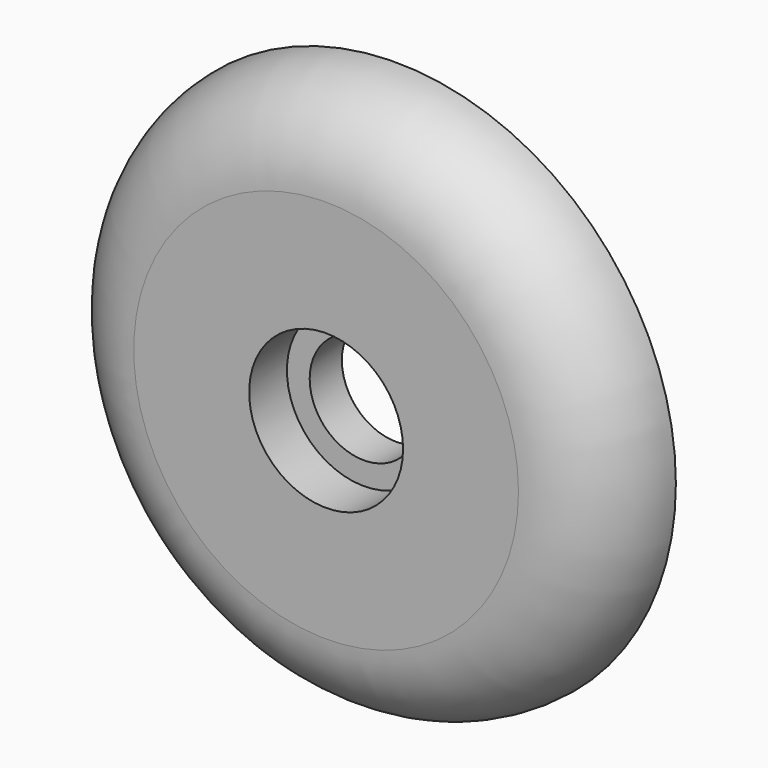
from build123d import *

# Parameters (mm, degrees)
F0_R     = 8
F1_DEPTH = 2.5
F2_R     = 2.49999
F3_R     = 1.55
F4_DEPTH = 25
F5_R     = 2.2
F5_R_2   = 1.55
F6_DEPTH = 1.35


# Not quite as in the source:
# - a fillet or chamfer is up to 0.001 mm smaller than in the source, because OpenCascade refuses the exact size


with BuildPart() as f1:
    # F0 (on Front) → F1 (new body)
    with BuildSketch(Plane.XZ):
        Circle(F0_R)
    extrude(amount=F1_DEPTH)

    # F2 (radius 2.5 in the source; OpenCascade refuses exactly that, so slightly less here)
    f2_edges = [f1.edges().sort_by_distance(p)[0] for p in [
        (-8, -2.5, 0),
    ]]
    fillet(f2_edges, radius=F2_R)

    # F3 (on face) → F4 (cut)
    with BuildSketch(Plane(origin=(0, 0, 0), x_dir=(-1, 0, 0), z_dir=(0, 1, 0))):
        Circle(F3_R)
    extrude(amount=-F4_DEPTH, mode=Mode.SUBTRACT)

    # F5 (on face) → F6 (cut)
    with BuildSketch(Plane.XZ.offset(2.5)):
        Circle(F5_R)
        Circle(F5_R_2, mode=Mode.SUBTRACT)
    extrude(amount=-F6_DEPTH, mode=Mode.SUBTRACT)


solid = f1.part
